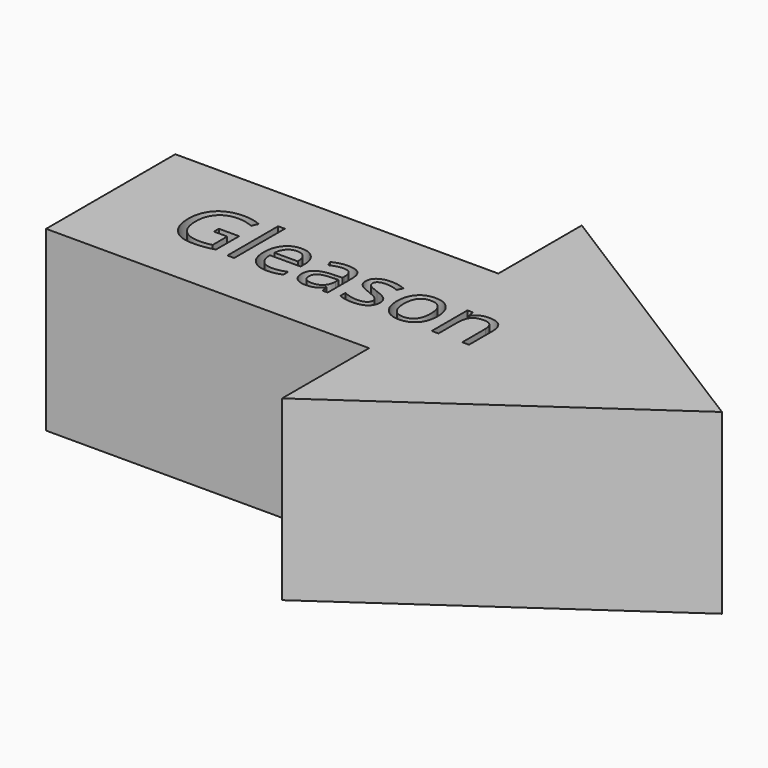
from build123d import *

# Parameters (mm, degrees)
F0_W         = 25.4
F0_H         = 12.7
F1_DEPTH     = 13.97
F2_TEXT_SIZE = 6.5534349738
F3_DEPTH     = 4.7625


# Not quite as in the source:
# - Text() gives the source's letters only with a copy of the font that has no kerning and outlines rounded to 1/6400 em; it was checked with that copy


with BuildPart() as f1:
    # F0 (on Top) → F1 (new body)
    with BuildSketch(Plane.XY):
        with Locations((-50.6003658891, 24.4945102095)):
            Rectangle(F0_W, F0_H)
        Polygon((-37.9003658891, 39.0487102095), (-37.9003658891, 30.8445102095), (-37.9003658891, 18.1445102095), (-37.9003658891, 9.593464516), (-15.6829096377, 25.0490866601), align=None)
    extrude(amount=F1_DEPTH)

    # F2 (on face) → F3 (cut)
    with BuildSketch(Plane.XY.offset(13.97)):
        with Locations((-57.7229186893, 22.3284102976)):
            Text('Gleason', F2_TEXT_SIZE, font='Open Sans', text_align=(TextAlign.LEFT, TextAlign.BOTTOM))
    extrude(amount=-F3_DEPTH, mode=Mode.SUBTRACT)


solid = f1.part
